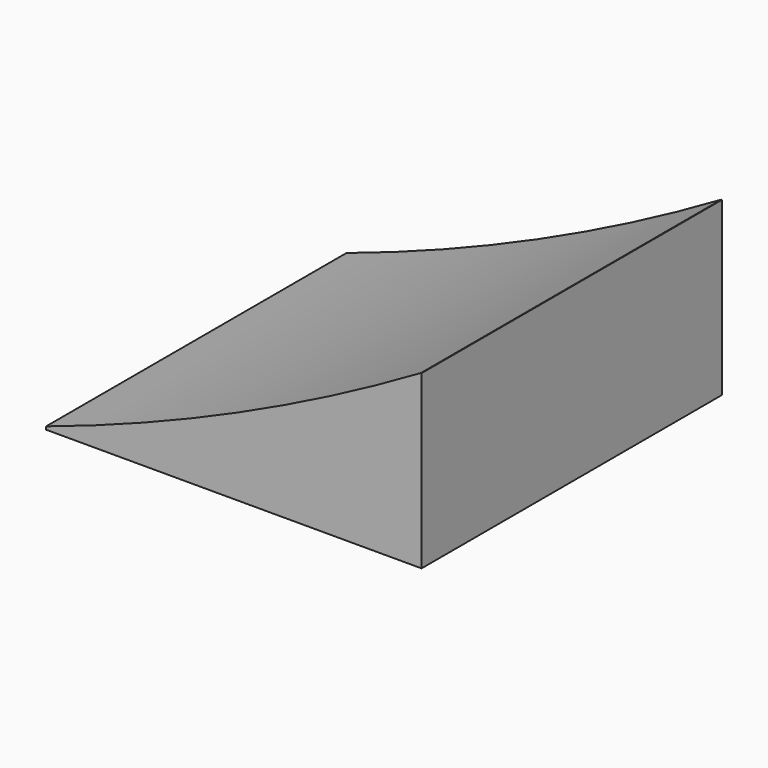
from build123d import *

# Parameters (mm, degrees)
F0_W     = 25.4
F0_H     = 11.6255704415
F1_DEPTH = 25.4
F3_DEPTH = 25.401


with BuildPart() as f1:
    # F0 (on Front) → F1 (new body)
    with BuildSketch(Plane.XZ):
        Rectangle(F0_W, F0_H)
    extrude(amount=F1_DEPTH)

    # F2 (on face) → F3 (cut, through all)
    with BuildSketch(Plane.XZ.offset(25.4)):
        with BuildLine():
            Line((-12.7, 5.8127852207), (-12.7, -5.613514744))
            ThreePointArc((-12.7, -5.613514744), (0.2798565548, -0.5667526673), (12.6591933696, 5.8127852207))
            Line((12.6591933696, 5.8127852207), (-12.7, 5.8127852207))
        make_face()
    extrude(amount=-F3_DEPTH, mode=Mode.SUBTRACT)


solid = f1.part
